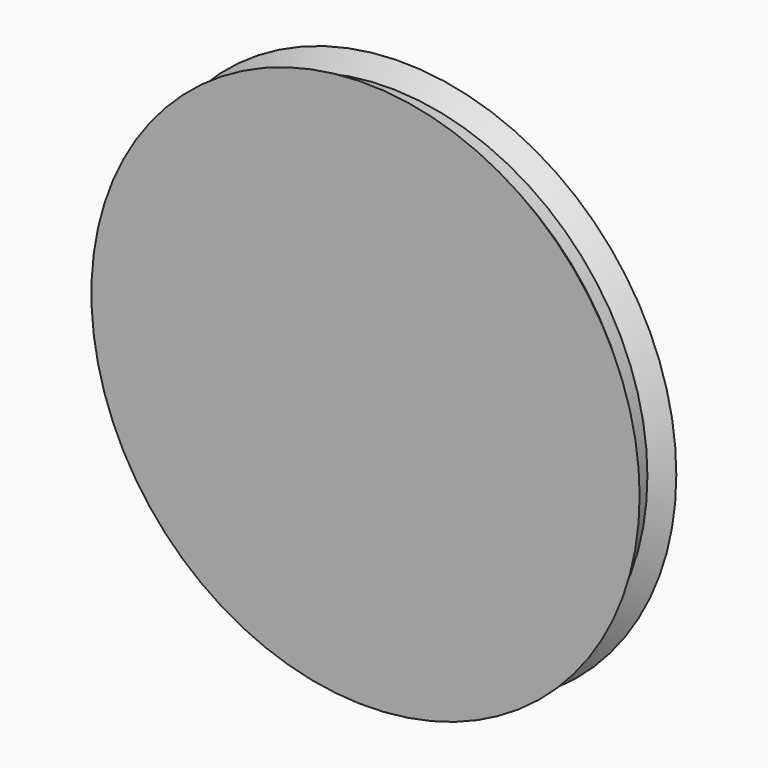
from build123d import *

# Parameters (mm, degrees)
F0_R     = 76.2
F1_DEPTH = 6.35
F2_R     = 76.2
F3_DEPTH = 1.5875
F4_R     = 71.4375
F5_DEPTH = 3.175


# Not quite as in the source:
# - a fillet or chamfer that OpenCascade refuses, or shapes differently, is made with other operations: its cross-section is extruded or revolved along the edge and cut away or added


with BuildPart() as f1:
    # F0 (on Front) → F1 (new body, symmetric)
    with BuildSketch(Plane.XZ):
        Circle(F0_R)
    extrude(amount=F1_DEPTH, both=True)

    # F2 (on Front) → F3 (cut, symmetric)
    with BuildSketch(Plane.XZ):
        Circle(F2_R)
    extrude(amount=F3_DEPTH, both=True, mode=Mode.SUBTRACT)

    # F6: chamfer of 5.08 on 1 edges, made by hand

    # F6_s1 → F6_t2 (revolve, cut)
    with BuildSketch(Plane.XY):
        Polygon((76.2, 6.6675), (71.12, 1.5875), (76.2, 1.5875), align=None)
    revolve(axis=Axis((0, 1.5875, 0), (0, -1, 0)), mode=Mode.SUBTRACT)

    # F6#s1: chamfer of 5.08 on 1 edges, made by hand

    # F6_s1_s1 → F6_s1_t2 (revolve, cut)
    with BuildSketch(Plane.XY):
        Polygon((76.2, -6.6675), (71.12, -1.5875), (76.2, -1.5875), align=None)
    revolve(axis=Axis((0, -1.5875, 0), (0, -1, 0)), mode=Mode.SUBTRACT)


with BuildPart() as f5:
    # F4 (on Front) → F5 (new body, symmetric)
    with BuildSketch(Plane.XZ):
        Circle(F4_R)
    extrude(amount=F5_DEPTH, both=True)


solid = Compound([f1.part, f5.part])
